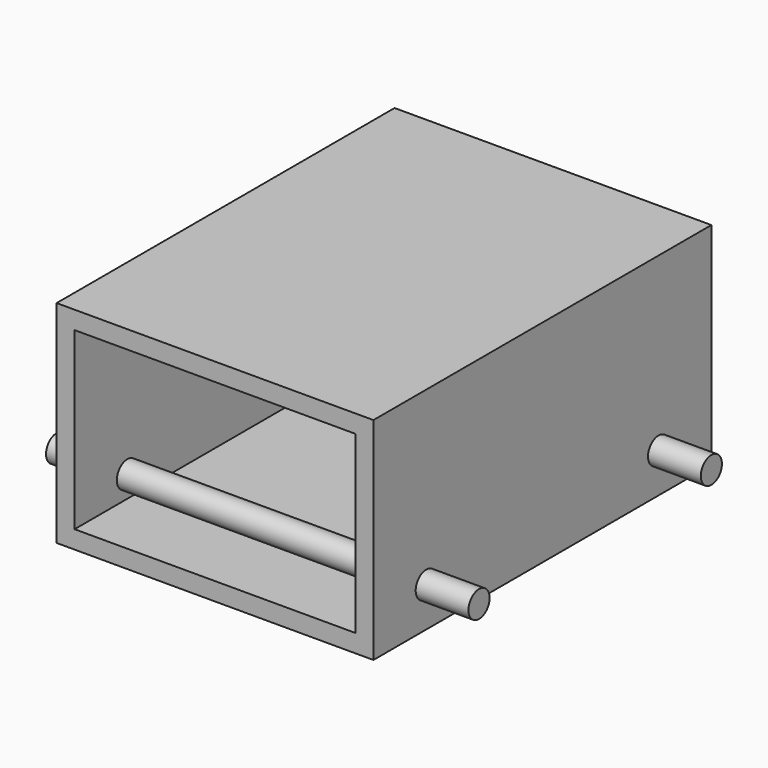
from build123d import *

# Parameters (mm, degrees)
F0_W     = 152.4
F0_H     = 101.6
F0_W_2   = 135.128
F0_H_2   = 84.328
F1_DEPTH = 101.6
F2_R     = 6.35
F3_DEPTH = 152.401
F4_R     = 6.35
F5_DEPTH = 101.6


with BuildPart() as f1:
    # F0 (on Front) → F1 (new body, symmetric)
    with BuildSketch(Plane.XZ):
        Rectangle(F0_W, F0_H)
        Rectangle(F0_W_2, F0_H_2, mode=Mode.SUBTRACT)
    extrude(amount=F1_DEPTH, both=True)

    # F2 (on face) → F3 (cut, through all)
    with BuildSketch(Plane.YZ.offset(76.2)):
        with Locations((-69.85, -31.75)):
            Circle(F2_R)
        with Locations((69.85, -31.75)):
            Circle(F2_R)
    extrude(amount=-F3_DEPTH, mode=Mode.SUBTRACT)


with BuildPart() as f5:
    # F4 (on Right) → F5 (new body, symmetric)
    with BuildSketch(Plane.YZ):
        with Locations((-69.85, -31.75)):
            Circle(F4_R)
    extrude(amount=F5_DEPTH, both=True)


with BuildPart() as f5b:
    # F4 (on Right) → F5, piece 2 (new body, symmetric)
    with BuildSketch(Plane.YZ):
        with Locations((69.85, -31.75)):
            Circle(F4_R)
    extrude(amount=F5_DEPTH, both=True)


solid = Compound([f1.part, f5.part, f5b.part])
